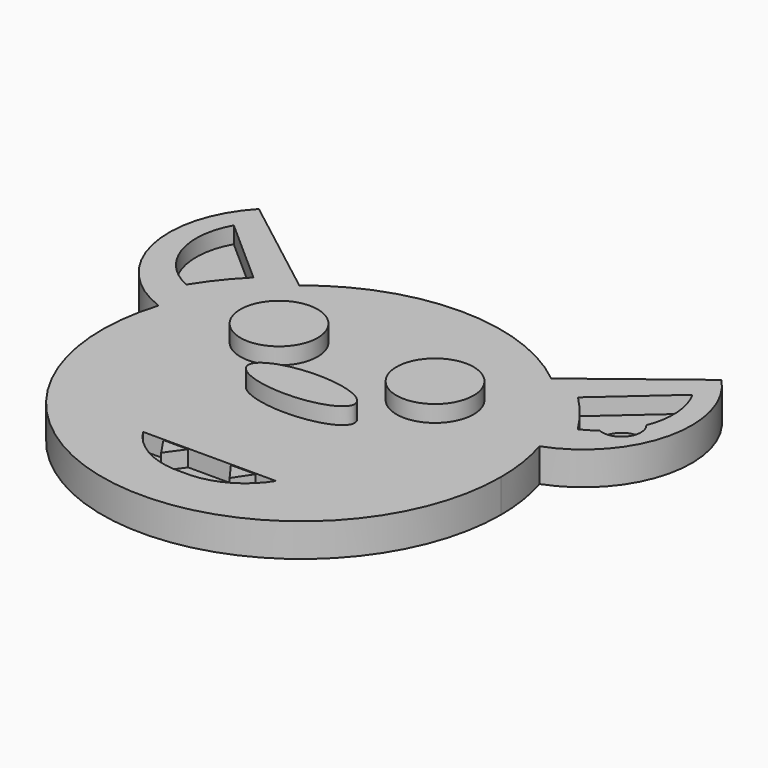
from build123d import *

# Parameters (mm, degrees)
F1_DEPTH  = 6.35
F3_DEPTH  = 3.175
F6_DEPTH  = 3.175
F8_DEPTH  = 3.175
F10_DEPTH = 3.048
F4_R      = 7.3778565178
F11_DEPTH = 3.175
F12_R     = 3.6859176852
F13_DEPTH = 6.351


# Not quite as in the source:
# - a feature names something its author has since deleted; it is built from what else it names


with BuildPart() as f1:
    # F0 (on Top) → F1 (new body)
    with BuildSketch(Plane.XY):
        with BuildLine():
            ThreePointArc((-36.3712396262, 11.3464940865), (-5.738718073, -37.6653304098), (38.1, 0))
            ThreePointArc((38.1, 0), (37.6653304098, 5.738718073), (36.3712396262, 11.3464940865))
            ThreePointArc((36.3712396262, 11.3464940865), (31.5544319278, 21.3524665018), (24.0569263159, 29.5444461148))
            ThreePointArc((24.0569263159, 29.5444461148), (0, 38.1), (-24.0569263159, 29.5444461148))
            ThreePointArc((-24.0569263159, 29.5444461148), (-31.5544319278, 21.3524665018), (-36.3712396262, 11.3464940865))
        make_face()
        with BuildLine():
            ThreePointArc((24.0569263159, 29.5444461148), (31.5544319278, 21.3524665018), (36.3712396262, 11.3464940865))
            ThreePointArc((36.3712396262, 11.3464940865), (49.3746579826, 26.088688726), (44.1774778249, 45.0468139009))
            Line((44.1774778249, 45.0468139009), (24.0569263159, 29.5444461148))
        make_face()
        with BuildLine():
            ThreePointArc((-44.1774778249, 45.0468139009), (-49.3746579826, 26.088688726), (-36.3712396262, 11.3464940865))
            ThreePointArc((-36.3712396262, 11.3464940865), (-31.5544319278, 21.3524665018), (-24.0569263159, 29.5444461148))
            Line((-24.0569263159, 29.5444461148), (-44.1774778249, 45.0468139009))
        make_face()
    extrude(amount=-F1_DEPTH)

    # F2 (on Top) → F3 (join)
    with BuildSketch(Plane.XY):
        with BuildLine():
            add(Edge.make_bspline(
                [(10.16, 0), (10.16, 6.7242064297), (-5.08, 3.3621032148), (-20.32, 0), (-5.08, -3.3621032148), (10.16, -6.7242064297), (10.16, 0)],
                knots=[0, 0, 0, 2.0943951024, 2.0943951024, 4.1887902048, 4.1887902048, 6.2831853072, 6.2831853072, 6.2831853072], degree=2, weights=[1, 0.5, 1, 0.5, 1, 0.5, 1]))
        make_face()
    extrude(amount=F3_DEPTH)

    # F5 (on face) → F6 (cut)
    with BuildSketch(Plane.XY):
        with BuildLine():
            Line((-30.9908390045, 27.2659789771), (-43.804358691, 38.5895557702))
            ThreePointArc((-43.804358691, 38.5895557702), (-44.8770730118, 27.4905174143), (-37.3975988477, 19.2202795297))
            ThreePointArc((-37.3975988477, 19.2202795297), (-34.4250124692, 23.4269092732), (-30.9908390045, 27.2659789771))
        make_face()
        with BuildLine():
            ThreePointArc((37.3975988477, 19.2202795297), (44.8770730118, 27.4905174143), (43.804358691, 38.5895557702))
            Line((43.804358691, 38.5895557702), (30.9908390045, 27.2659789771))
            ThreePointArc((30.9908390045, 27.2659789771), (34.4250124692, 23.4269092732), (37.3975988477, 19.2202795297))
        make_face()
    extrude(amount=-F6_DEPTH, mode=Mode.SUBTRACT)

    # F7 (on face) → F8 (cut)
    with BuildSketch(Plane.XY):
        with BuildLine():
            Line((12.7, -21.9528563652), (0, -21.9528563652))
            Line((0, -21.9528563652), (-12.7, -21.9528563652))
            ThreePointArc((-12.7, -21.9528563652), (-7.2401700339, -26.9432924529), (0, -28.4579321742))
            ThreePointArc((0, -28.4579321742), (7.2401700339, -26.9432924529), (12.7, -21.9528563652))
        make_face()
    extrude(amount=-F8_DEPTH, mode=Mode.SUBTRACT)

    # F9 (on face) → F10 (join)
    with BuildSketch(Plane.XY.offset(-3.175)):
        Polygon((-4.0704635903, -21.9528563652), (-8.815612644, -21.9528563652), (-6.5379412845, -25.3327768296), align=None)
        Polygon((4.0704635903, -21.9528563652), (6.5379412845, -25.3327768296), (8.815612644, -21.9528563652), align=None)
    extrude(amount=F10_DEPTH)

    # F4 (on face) → F11 (join)
    with BuildSketch(Plane.XY):
        with Locations((-14.8994419724, 13.2605032995)):
            Circle(F4_R)
        with Locations((14.8994419724, 13.2605032995)):
            Circle(F4_R)
    extrude(amount=F11_DEPTH)

    # F12 (on face) → F13 (cut, through all)
    with BuildSketch(Plane.XY):
        with Locations((41.7184382677, 24.286089465)):
            Circle(F12_R)
    extrude(amount=-F13_DEPTH, mode=Mode.SUBTRACT)


solid = f1.part
